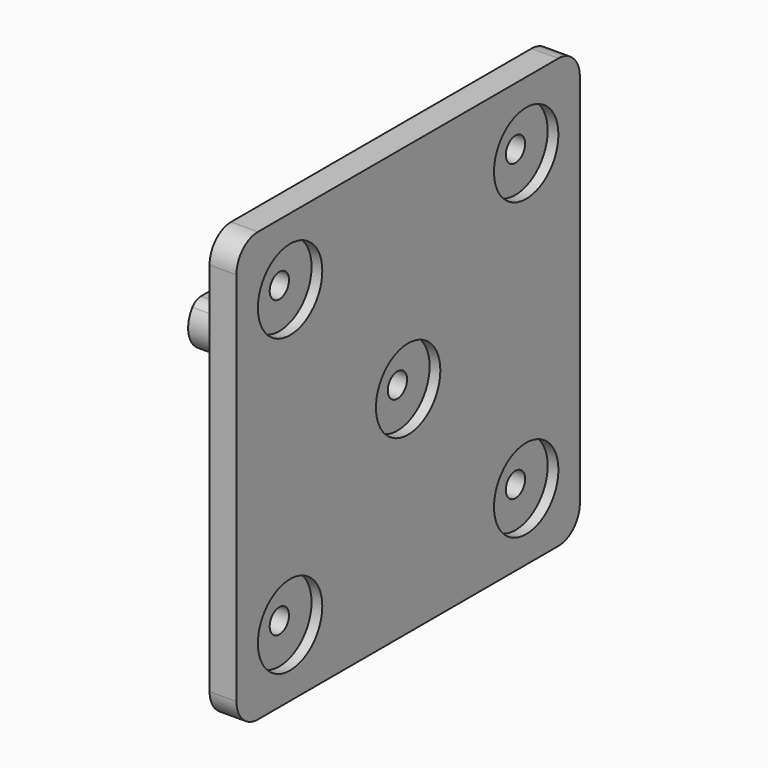
from build123d import *

# Parameters (mm, degrees)
F1_R            = 27.5
F2_DEPTH        = 5
F3_W            = 80
F3_H            = 80
F3_R            = 27.5
F4_DEPTH        = 5
F5_DEPTH        = 2
F6_R            = 4
F7_R            = 1
F8_R            = 0.25
F9_R            = 11
F9_R_2          = 8
F10_DEPTH       = 10
F11_DEPTH       = 17
F13_DEPTH       = 10
F15_D           = 4.5
F15_CBORE_D     = 15
F15_CBORE_DEPTH = 2
F16_R           = 5
F17_R           = 2.5
F18_R           = 0.2


with BuildPart() as f2:
    # F1 (on Right) → F2 (new body)
    with BuildSketch(Plane.YZ):
        Circle(F1_R)
    extrude(amount=F2_DEPTH)

    # F3 (on face) → F4 (join)
    with BuildSketch(Plane.YZ.offset(5)):
        Rectangle(F3_W, F3_H)
        Circle(F3_R, mode=Mode.SUBTRACT)
        Circle(F3_R)
    extrude(amount=F4_DEPTH)

    # F0 (on Right) → F5 (cut)
    with BuildSketch(Plane.YZ):
        with BuildLine():
            ThreePointArc((-23.6643191324, 4), (-21.8753683688, 6.2092535777), (-19.8809679086, 8.2349665408))
            ThreePointArc((-19.8809679086, 8.2349665408), (-19.8588266254, 11.0776160037), (-19.5616276554, 13.9047734059))
            ThreePointArc((-19.5616276554, 13.9047734059), (-22.1731087803, 9.1844023768), (-23.6643191324, 4))
        make_face()
        with BuildLine():
            ThreePointArc((-18.3487984588, 0), (-19.145364712, 2.7946820532), (-19.6614989956, 5.6544671806))
            ThreePointArc((-19.6614989956, 5.6544671806), (-21.943993508, 2.963054611), (-23.8607068909, 0))
            ThreePointArc((-23.8607068909, 0), (-21.943993508, -2.963054611), (-19.6614989956, -5.6544671806))
            ThreePointArc((-19.6614989956, -5.6544671806), (-19.145364712, -2.7946820532), (-18.3487984588, 0))
        make_face()
        with BuildLine():
            ThreePointArc((-11.2901120254, 9.8758984631), (-15.1560824108, 9.1425557797), (-18.8590982257, 7.8116942592))
            ThreePointArc((-18.8590982257, 7.8116942592), (-17.1817318382, 4.2522054597), (-14.9666295471, 1))
            ThreePointArc((-14.9666295471, 1), (-13.8581929877, 5.7402514855), (-11.2901120254, 9.8758984631))
        make_face()
        with BuildLine():
            ThreePointArc((-9.9044671806, 17.9010913555), (-13.4215506074, 17.6119426243), (-16.8720676465, 16.8720676465))
            ThreePointArc((-16.8720676465, 16.8720676465), (-17.6119426243, 13.4215506074), (-17.9010913555, 9.9044671806))
            ThreePointArc((-17.9010913555, 9.9044671806), (-15.5139558472, 11.561678585), (-12.9745598169, 12.9745598169))
            ThreePointArc((-12.9745598169, 12.9745598169), (-11.561678585, 15.5139558472), (-9.9044671806, 17.9010913555))
        make_face()
        with BuildLine():
            ThreePointArc((-8.2349665408, 19.8809679086), (-6.2092535777, 21.8753683688), (-4, 23.6643191324))
            ThreePointArc((-4, 23.6643191324), (-9.1844023768, 22.1731087803), (-13.9047734059, 19.5616276554))
            ThreePointArc((-13.9047734059, 19.5616276554), (-11.0776160037, 19.8588266254), (-8.2349665408, 19.8809679086))
        make_face()
        with BuildLine():
            ThreePointArc((-9.8758984631, 11.2901120254), (-5.7402514855, 13.8581929877), (-1, 14.9666295471))
            ThreePointArc((-1, 14.9666295471), (-4.2522054597, 17.1817318382), (-7.8116942592, 18.8590982257))
            ThreePointArc((-7.8116942592, 18.8590982257), (-9.1425557797, 15.1560824108), (-9.8758984631, 11.2901120254))
        make_face()
        with BuildLine():
            ThreePointArc((5.6544671806, 19.6614989956), (2.963054611, 21.943993508), (0, 23.8607068909))
            ThreePointArc((0, 23.8607068909), (-2.963054611, 21.943993508), (-5.6544671806, 19.6614989956))
            ThreePointArc((-5.6544671806, 19.6614989956), (-2.7946820532, 19.145364712), (0, 18.3487984588))
            ThreePointArc((0, 18.3487984588), (2.7946820532, 19.145364712), (5.6544671806, 19.6614989956))
        make_face()
        with BuildLine():
            ThreePointArc((4, 23.6643191324), (6.2092535777, 21.8753683688), (8.2349665408, 19.8809679086))
            ThreePointArc((8.2349665408, 19.8809679086), (11.0776160037, 19.8588266254), (13.9047734059, 19.5616276554))
            ThreePointArc((13.9047734059, 19.5616276554), (9.1844023768, 22.1731087803), (4, 23.6643191324))
        make_face()
        with BuildLine():
            ThreePointArc((9.8758984631, 11.2901120254), (9.1425557797, 15.1560824108), (7.8116942592, 18.8590982257))
            ThreePointArc((7.8116942592, 18.8590982257), (4.2522054597, 17.1817318382), (1, 14.9666295471))
            ThreePointArc((1, 14.9666295471), (5.7402514855, 13.8581929877), (9.8758984631, 11.2901120254))
        make_face()
        with BuildLine():
            ThreePointArc((17.9010913555, 9.9044671806), (17.6119426243, 13.4215506074), (16.8720676465, 16.8720676465))
            ThreePointArc((16.8720676465, 16.8720676465), (13.4215506074, 17.6119426243), (9.9044671806, 17.9010913555))
            ThreePointArc((9.9044671806, 17.9010913555), (11.561678585, 15.5139558472), (12.9745598169, 12.9745598169))
            ThreePointArc((12.9745598169, 12.9745598169), (15.5139558472, 11.561678585), (17.9010913555, 9.9044671806))
        make_face()
        with BuildLine():
            ThreePointArc((19.5616276554, 13.9047734059), (19.8588266254, 11.0776160037), (19.8809679086, 8.2349665408))
            ThreePointArc((19.8809679086, 8.2349665408), (21.8753683688, 6.2092535777), (23.6643191324, 4))
            ThreePointArc((23.6643191324, 4), (22.1731087803, 9.1844023768), (19.5616276554, 13.9047734059))
        make_face()
        with BuildLine():
            ThreePointArc((11.2901120254, 9.8758984631), (13.8581929877, 5.7402514855), (14.9666295471, 1))
            ThreePointArc((14.9666295471, 1), (17.1817318382, 4.2522054597), (18.8590982257, 7.8116942592))
            ThreePointArc((18.8590982257, 7.8116942592), (15.1560824108, 9.1425557797), (11.2901120254, 9.8758984631))
        make_face()
        with BuildLine():
            ThreePointArc((19.6614989956, -5.6544671806), (21.943993508, -2.963054611), (23.8607068909, 0))
            ThreePointArc((23.8607068909, 0), (21.943993508, 2.963054611), (19.6614989956, 5.6544671806))
            ThreePointArc((19.6614989956, 5.6544671806), (19.145364712, 2.7946820532), (18.3487984588, 0))
            ThreePointArc((18.3487984588, 0), (19.145364712, -2.7946820532), (19.6614989956, -5.6544671806))
        make_face()
        with BuildLine():
            ThreePointArc((11.2901120254, -9.8758984631), (15.1560824108, -9.1425557797), (18.8590982257, -7.8116942592))
            ThreePointArc((18.8590982257, -7.8116942592), (17.1817318382, -4.2522054597), (14.9666295471, -1))
            ThreePointArc((14.9666295471, -1), (13.8581929877, -5.7402514855), (11.2901120254, -9.8758984631))
        make_face()
        with BuildLine():
            ThreePointArc((17.9010913555, -9.9044671806), (15.5139558472, -11.561678585), (12.9745598169, -12.9745598169))
            ThreePointArc((12.9745598169, -12.9745598169), (11.561678585, -15.5139558472), (9.9044671806, -17.9010913555))
            ThreePointArc((9.9044671806, -17.9010913555), (13.4215506074, -17.6119426243), (16.8720676465, -16.8720676465))
            ThreePointArc((16.8720676465, -16.8720676465), (17.6119426243, -13.4215506074), (17.9010913555, -9.9044671806))
        make_face()
        with BuildLine():
            ThreePointArc((23.6643191324, -4), (21.8753683688, -6.2092535777), (19.8809679086, -8.2349665408))
            ThreePointArc((19.8809679086, -8.2349665408), (19.8588266254, -11.0776160037), (19.5616276554, -13.9047734059))
            ThreePointArc((19.5616276554, -13.9047734059), (22.1731087803, -9.1844023768), (23.6643191324, -4))
        make_face()
        with BuildLine():
            ThreePointArc((8.2349665408, -19.8809679086), (6.2092535777, -21.8753683688), (4, -23.6643191324))
            ThreePointArc((4, -23.6643191324), (9.1844023768, -22.1731087803), (13.9047734059, -19.5616276554))
            ThreePointArc((13.9047734059, -19.5616276554), (11.0776160037, -19.8588266254), (8.2349665408, -19.8809679086))
        make_face()
        with BuildLine():
            ThreePointArc((9.8758984631, -11.2901120254), (5.7402514855, -13.8581929877), (1, -14.9666295471))
            ThreePointArc((1, -14.9666295471), (4.2522054597, -17.1817318382), (7.8116942592, -18.8590982257))
            ThreePointArc((7.8116942592, -18.8590982257), (9.1425557797, -15.1560824108), (9.8758984631, -11.2901120254))
        make_face()
        with BuildLine():
            ThreePointArc((0, -18.3487984588), (-2.7946820532, -19.145364712), (-5.6544671806, -19.6614989956))
            ThreePointArc((-5.6544671806, -19.6614989956), (-2.963054611, -21.943993508), (0, -23.8607068909))
            ThreePointArc((0, -23.8607068909), (2.963054611, -21.943993508), (5.6544671806, -19.6614989956))
            ThreePointArc((5.6544671806, -19.6614989956), (2.7946820532, -19.145364712), (0, -18.3487984588))
        make_face()
        with BuildLine():
            ThreePointArc((-1, -14.9666295471), (-5.7402514855, -13.8581929877), (-9.8758984631, -11.2901120254))
            ThreePointArc((-9.8758984631, -11.2901120254), (-9.1425557797, -15.1560824108), (-7.8116942592, -18.8590982257))
            ThreePointArc((-7.8116942592, -18.8590982257), (-4.2522054597, -17.1817318382), (-1, -14.9666295471))
        make_face()
        with BuildLine():
            ThreePointArc((-8.2349665408, -19.8809679086), (-11.0776160037, -19.8588266254), (-13.9047734059, -19.5616276554))
            ThreePointArc((-13.9047734059, -19.5616276554), (-9.1844023768, -22.1731087803), (-4, -23.6643191324))
            ThreePointArc((-4, -23.6643191324), (-6.2092535777, -21.8753683688), (-8.2349665408, -19.8809679086))
        make_face()
        with BuildLine():
            ThreePointArc((-12.9745598169, -12.9745598169), (-15.5139558472, -11.561678585), (-17.9010913555, -9.9044671806))
            ThreePointArc((-17.9010913555, -9.9044671806), (-17.6119426243, -13.4215506074), (-16.8720676465, -16.8720676465))
            ThreePointArc((-16.8720676465, -16.8720676465), (-13.4215506074, -17.6119426243), (-9.9044671806, -17.9010913555))
            ThreePointArc((-9.9044671806, -17.9010913555), (-11.561678585, -15.5139558472), (-12.9745598169, -12.9745598169))
        make_face()
        with BuildLine():
            ThreePointArc((-19.8809679086, -8.2349665408), (-21.8753683688, -6.2092535777), (-23.6643191324, -4))
            ThreePointArc((-23.6643191324, -4), (-22.1731087803, -9.1844023768), (-19.5616276554, -13.9047734059))
            ThreePointArc((-19.5616276554, -13.9047734059), (-19.8588266254, -11.0776160037), (-19.8809679086, -8.2349665408))
        make_face()
        with BuildLine():
            ThreePointArc((-11.2901120254, -9.8758984631), (-13.8581929877, -5.7402514855), (-14.9666295471, -1))
            ThreePointArc((-14.9666295471, -1), (-17.1817318382, -4.2522054597), (-18.8590982257, -7.8116942592))
            ThreePointArc((-18.8590982257, -7.8116942592), (-15.1560824108, -9.1425557797), (-11.2901120254, -9.8758984631))
        make_face()
    extrude(amount=F5_DEPTH, mode=Mode.SUBTRACT)

    # F6
    f6_edges = [f2.edges().sort_by_distance(p)[0] for p in [
        (1, 18.859098, 7.811694),
        (1, 19.880968, 8.234967),
        (1, 8.234967, 19.880968),
        (1, 7.811694, 18.859098),
        (1, -7.811694, 18.859098),
        (1, -8.234967, 19.880968),
        (1, -19.880968, 8.234967),
        (1, -18.859098, 7.811694),
        (1, -18.859098, -7.811694),
        (1, -19.880968, -8.234967),
        (1, -7.811694, -18.859098),
        (1, -8.234967, -19.880968),
        (1, 7.811694, -18.859098),
        (1, 8.234967, -19.880968),
        (1, 19.880968, -8.234967),
        (1, 18.859098, -7.811694),
        (1, 18.348798, 0),
        (1, 23.860707, 0),
        (1, 16.872068, -16.872068),
        (1, 12.97456, -12.97456),
        (1, 0, -18.348798),
        (1, 0, -23.860707),
        (1, -16.872068, -16.872068),
        (1, -12.97456, -12.97456),
        (1, -18.348798, 0),
        (1, -23.860707, 0),
        (1, -16.872068, 16.872068),
        (1, -12.97456, 12.97456),
        (1, 0, 18.348798),
        (1, 0, 23.860707),
        (1, 12.97456, 12.97456),
        (1, 16.872068, 16.872068),
    ]]
    fillet(f6_edges, radius=F6_R)

    # F7
    f7_edges = [f2.edges().sort_by_distance(p)[0] for p in [
        (1, 14.96663, -1),
        (1, 14.96663, 1),
        (1, 11.290112, 9.875898),
        (1, 9.875898, 11.290112),
        (1, 1, 14.96663),
        (1, -1, 14.96663),
        (1, -9.875898, 11.290112),
        (1, -11.290112, 9.875898),
        (1, -14.96663, 1),
        (1, -14.96663, -1),
        (1, -11.290112, -9.875898),
        (1, -9.875898, -11.290112),
        (1, -1, -14.96663),
        (1, 1, -14.96663),
        (1, 9.875898, -11.290112),
        (1, 11.290112, -9.875898),
    ]]
    fillet(f7_edges, radius=F7_R)

    # F8
    f8_edges = [f2.edges().sort_by_distance(p)[0] for p in [
        (1, 9.904467, 17.901091),
        (1, 4, 23.664319),
        (1, 13.904773, 19.561628),
        (1, 5.654467, 19.661499),
        (1, -5.654467, 19.661499),
        (1, -13.904773, 19.561628),
        (1, -4, 23.664319),
        (1, -9.904467, 17.901091),
        (1, -17.901091, 9.904467),
        (1, -23.664319, 4),
        (1, -19.561628, 13.904773),
        (1, -19.661499, 5.654467),
        (1, -19.661499, -5.654467),
        (1, -19.561628, -13.904773),
        (1, -23.664319, -4),
        (1, -17.901091, -9.904467),
        (1, -9.904467, -17.901091),
        (1, -4, -23.664319),
        (1, -13.904773, -19.561628),
        (1, -5.654467, -19.661499),
        (1, 5.654467, -19.661499),
        (1, 4, -23.664319),
        (1, 13.904773, -19.561628),
        (1, 9.904467, -17.901091),
        (1, 17.901091, -9.904467),
        (1, 19.561628, -13.904773),
        (1, 23.664319, -4),
        (1, 19.661499, -5.654467),
        (1, 19.661499, 5.654467),
        (1, 19.561628, 13.904773),
        (1, 23.664319, 4),
        (1, 17.901091, 9.904467),
    ]]
    fillet(f8_edges, radius=F8_R)

    # F9 (on face) → F10 (join)
    with BuildSketch(Plane(origin=(0, 0, 0), x_dir=(0, -1, 0), z_dir=(-1, 0, 0))):
        Circle(F9_R)
        Circle(F9_R_2, mode=Mode.SUBTRACT)
    extrude(amount=F10_DEPTH)

    # F11 (add): a face of the model
    f11_faces = [f2.faces().sort_by_distance(p)[0] for p in [
        (0, 0, 0),
    ]]
    extrude(f11_faces, amount=F11_DEPTH)

    # F12 (on face) → F13 (join)
    with BuildSketch(Plane(origin=(-17, 0, 0), x_dir=(0, -1, 0), z_dir=(-1, 0, 0))):
        with BuildLine():
            ThreePointArc((-3, 4), (-2.2360679775, -4.472135955), (5, 0))
            ThreePointArc((5, 0), (4.472135955, 2.2360679775), (3, 4))
            Line((3, 4), (-3, 4))
        make_face()
    extrude(amount=F13_DEPTH)

    # F15 (through all)
    with Locations(Plane.YZ.offset(10)):
        with Locations((-27.5, 27.5), (-27.5, -27.5), (27.5, 27.5), (27.5, -27.5), (0, 0)):
            CounterBoreHole(F15_D / 2, F15_CBORE_D / 2, F15_CBORE_DEPTH)

    # F16
    f16_edges = [f2.edges().sort_by_distance(p)[0] for p in [
        (7.5, 40, 40),
        (7.5, -40, 40),
        (7.5, -40, -40),
        (7.5, 40, -40),
    ]]
    fillet(f16_edges, radius=F16_R)

    # F17
    f17_edges = [f2.edges().sort_by_distance(p)[0] for p in [
        (-22, 3, 4),
        (-22, -3, 4),
    ]]
    fillet(f17_edges, radius=F17_R)

    # F18
    f18_edges = [f2.edges().sort_by_distance(p)[0] for p in [
        (-10, 11, 0),
    ]]
    fillet(f18_edges, radius=F18_R)


solid = f2.part
